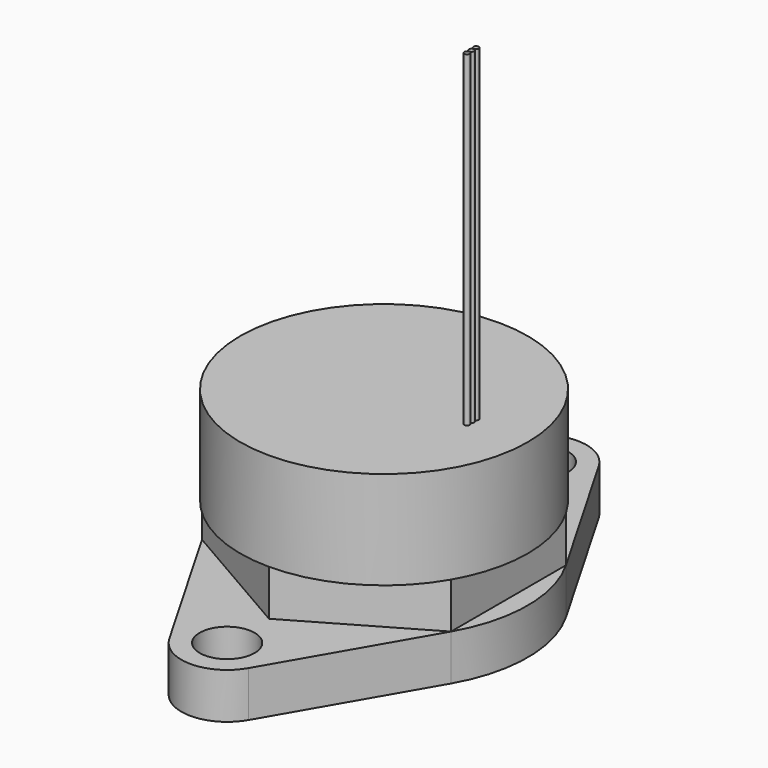
from build123d import *

# Parameters (mm, degrees)
F0_R      = 11
F1_DEPTH  = 14.5
F2_R      = 2.1
F3_DEPTH  = 3.5
F4_R      = 11
F5_DEPTH  = 3.5
F7_DEPTH  = 3.5
F8_R      = 6.5
F9_DEPTH  = 7.34
F10_R     = 0.2032
F11_DEPTH = 25


# Not quite as in the source:
# - a pattern or mirror of a feature is missing from the dataset's text; its kind, count and spacing are read off the source's solid


with BuildPart() as f1:
    # F0 (on Top) → F1 (new body)
    with BuildSketch(Plane.XY):
        Circle(F0_R)
    extrude(amount=F1_DEPTH)

    # F2 (on face) → F3 (join)
    with BuildSketch(Plane(origin=(0, 0, 0), x_dir=(1, 0, 0), z_dir=(0, 0, -1))):
        with BuildLine():
            Line((9.5262794416, 5.5), (3.0310889132, 16.75))
            ThreePointArc((3.0310889132, 16.75), (0, 18.5), (-3.0310889132, 16.75))
            Line((-3.0310889132, 16.75), (-9.5262794416, 5.5))
            ThreePointArc((-9.5262794416, 5.5), (0, 11), (9.5262794416, 5.5))
        make_face()
        with Locations((0, 15)):
            Circle(F2_R, mode=Mode.SUBTRACT)
        with BuildLine():
            ThreePointArc((9.5262794416, -5.5), (0, -11), (-9.5262794416, -5.5))
            Line((-9.5262794416, -5.5), (-3.0310889132, -16.75))
            ThreePointArc((-3.0310889132, -16.75), (0, -18.5), (3.0310889132, -16.75))
            Line((3.0310889132, -16.75), (9.5262794416, -5.5))
        make_face()
        with Locations((0, -15)):
            Circle(F2_R, mode=Mode.SUBTRACT)
    f3 = extrude(amount=-F3_DEPTH)

    # F3_copies: F3 across plane
    add(f3.mirror(Plane(origin=(0, 0, 0), x_dir=(0, 0, -1), z_dir=(-1, 0, 0))))

    # F4 (on face) → F5 (cut)
    with BuildSketch(Plane.XY.offset(3.5)):
        Circle(F4_R)
    extrude(amount=F5_DEPTH, mode=Mode.SUBTRACT)

    # F6 (on face) → F7 (join)
    with BuildSketch(Plane.XY.offset(3.5)):
        Polygon((9.5262794416, 5.5), (0, 11), (-9.5262794416, 5.5), (-9.5262794416, -5.5), (0, -11), (9.5262794416, -5.5), align=None)
    extrude(amount=F7_DEPTH)

    # F8 (on face) → F9 (cut)
    with BuildSketch(Plane(origin=(0, 0, 0), x_dir=(1, 0, 0), z_dir=(0, 0, -1))):
        Circle(F8_R)
    extrude(amount=-F9_DEPTH, mode=Mode.SUBTRACT)

    # F10 (on face) → F11 (join)
    with BuildSketch(Plane.XY.offset(14.5)):
        with Locations((6.7, 0)):
            Circle(F10_R)
        with Locations((6.7, 0.4318)):
            Circle(F10_R)
        with Locations((6.7, -0.4318)):
            Circle(F10_R)
    extrude(amount=F11_DEPTH)


solid = f1.part
